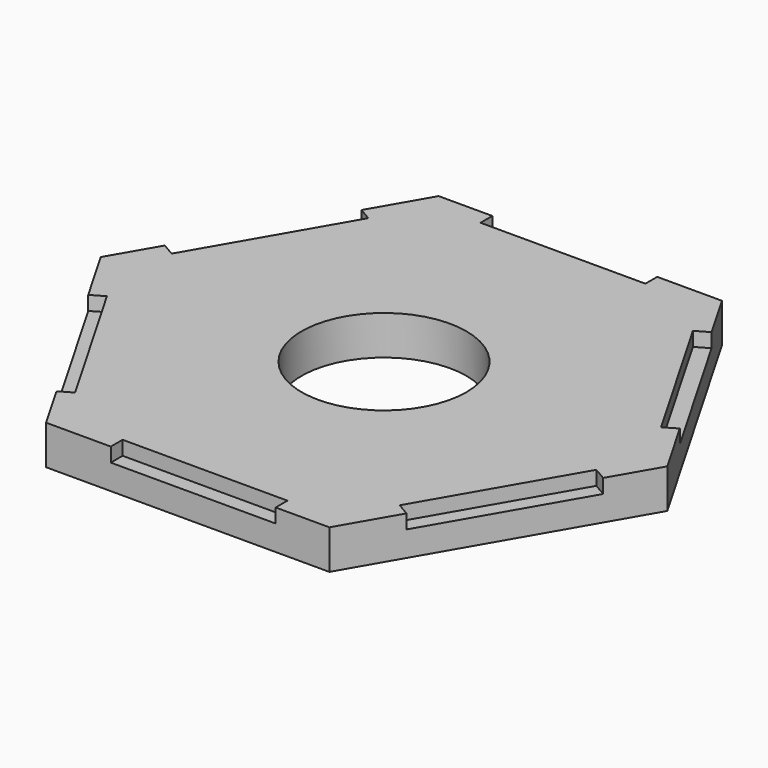
from build123d import *

# Parameters (mm, degrees)
F1_DEPTH        = 6.35
F2_R            = 13.335
F3_DEPTH        = 25.4
F5_DEPTH        = 2.286
F5_COPIES_COUNT = 6


# Not quite as in the source:
# - a pattern or mirror of a feature is missing from the dataset's text; its kind, count and spacing are read off the source's solid


with BuildPart() as f1:
    # F0 (on Top) → F1 (new body)
    with BuildSketch(Plane.XY):
        Polygon((22.9135888085, 39.6875), (-22.9135888085, 39.6875), (-45.8271776169, 0), (-22.9135888085, -39.6875), (22.9135888085, -39.6875), (45.8271776169, 0), align=None)
    extrude(amount=F1_DEPTH)

    # F2 (on face) → F3 (cut)
    with BuildSketch(Plane.XY.offset(6.35)):
        Circle(F2_R)
    extrude(amount=-F3_DEPTH, mode=Mode.SUBTRACT)

    # F4 (on face) → F5 (cut)
    with BuildSketch(Plane.XY.offset(6.35)):
        Polygon((-38.5256609586, -7.8713978245), (-40.5933832127, -9.0651978245), (-27.2583832127, -32.1620953434), (-25.1906609586, -30.9682953434), align=None)
    f5 = extrude(amount=-F5_DEPTH, mode=Mode.SUBTRACT)

    # F5_copies: F5 ×6 about axis
    f5_copies_axis = Axis((0, 0, 0), (0, 0, 1))
    for i in range(1, F5_COPIES_COUNT):
        add(f5.rotate(f5_copies_axis, i * 360 / F5_COPIES_COUNT), mode=Mode.SUBTRACT)


solid = f1.part
